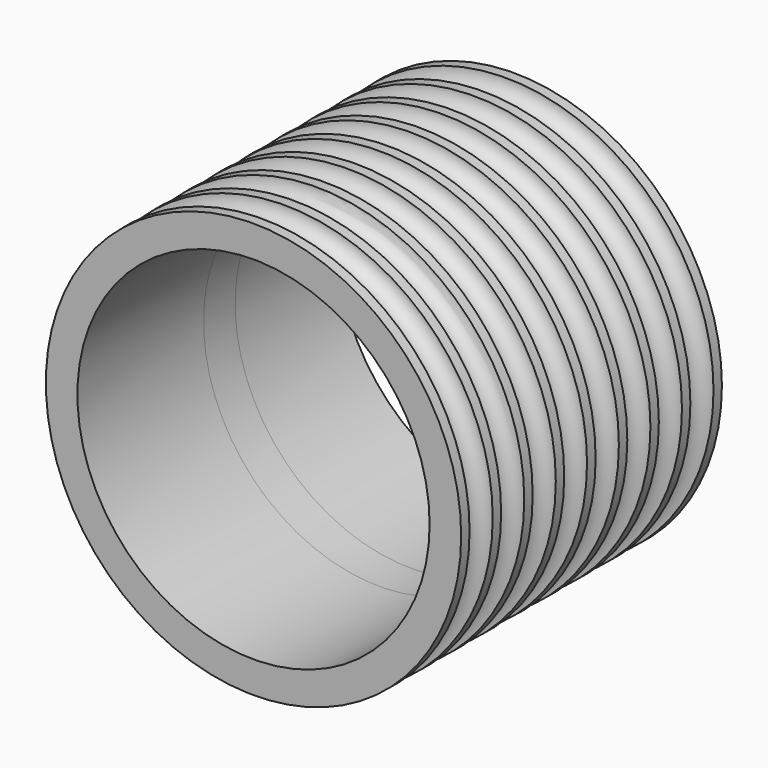
from build123d import *


# Not quite as in the source:
# - a feature names something its author has since deleted; it is built from what else it names


with BuildPart() as f1:
    # F0 (on Top) → F1 (revolve)
    with BuildSketch(Plane.XY):
        with BuildLine():
            Line((19.7205603719, 0.4943568721), (16.75, 0.4943568721))
            Line((16.75, 0.4943568721), (16.75, 0))
            Line((16.75, 0), (16.75, -2.2556431279))
            Line((16.75, -2.2556431279), (19.6911373127, -2.2556431279))
            ThreePointArc((19.6911373127, -2.2556431279), (18.3454816726, -0.8660881593), (19.7205603719, 0.4943568721))
        make_face()
        with BuildLine():
            Line((16.7490182523, 4.2443567436), (16.75, 0.4943568721))
            Line((16.75, 0.4943568721), (19.7205603719, 0.4943568721))
            Line((19.7205603719, 0.4943568721), (19.7389115558, 1.4941884749))
            ThreePointArc((19.7389115558, 1.4941884749), (18.3735909849, 2.8624558945), (19.7251108834, 4.2443567436))
            Line((19.7251108834, 4.2443567436), (16.7490182523, 4.2443567436))
        make_face()
        with BuildLine():
            Line((16.7490182523, 7.9943567436), (16.7490182523, 4.2443567436))
            Line((16.7490182523, 4.2443567436), (19.7251108834, 4.2443567436))
            ThreePointArc((19.7251108834, 4.2443567436), (19.7369436677, 4.244509486), (19.7487773282, 4.2445604014))
            Line((19.7487773282, 4.2445604014), (19.7487773282, 5.2443567436))
            ThreePointArc((19.7487773282, 5.2443567436), (18.3737773282, 6.6193567436), (19.7487773282, 7.9943567436))
            Line((19.7487773282, 7.9943567436), (16.7490182523, 7.9943567436))
        make_face()
        with BuildLine():
            Line((19.6911373127, -2.2556431279), (16.75, -2.2556431279))
            Line((16.75, -2.2556431279), (16.75, -6.0056431279))
            Line((16.75, -6.0056431279), (19.7499834311, -6.0056431279))
            ThreePointArc((19.7499834311, -6.0056431279), (18.3969368426, -4.6306431279), (19.7499834311, -3.2556431279))
            Line((19.7499834311, -3.2556431279), (19.7499834311, -2.2556431279))
            ThreePointArc((19.7499834311, -2.2556431279), (19.7205603719, -2.2559579339), (19.6911373127, -2.2556431279))
        make_face()
        with BuildLine():
            Line((19.7499834311, -2.2556431279), (19.6911373127, -2.2556431279))
            ThreePointArc((19.6911373127, -2.2556431279), (19.7205603719, -2.2559579339), (19.7499834311, -2.2556431279))
        make_face()
        with BuildLine():
            ThreePointArc((19.7487773282, 4.2445604014), (19.7369436677, 4.244509486), (19.7251108834, 4.2443567436))
            Line((19.7251108834, 4.2443567436), (19.7487773282, 4.2443567436))
            Line((19.7487773282, 4.2443567436), (19.7487773282, 4.2445604014))
        make_face()
        with BuildLine():
            Line((16.7490182523, 11.7443567436), (16.7490182523, 7.9943567436))
            Line((16.7490182523, 7.9943567436), (19.7487773282, 7.9943567436))
            Line((19.7487773282, 7.9943567436), (19.7487773282, 8.9943567436))
            ThreePointArc((19.7487773282, 8.9943567436), (18.3737773282, 10.3693567436), (19.7487773282, 11.7443567436))
            Line((19.7487773282, 11.7443567436), (16.7490182523, 11.7443567436))
        make_face()
        with BuildLine():
            Line((19.7499834311, -6.0056431279), (16.75, -6.0056431279))
            Line((16.75, -6.0056431279), (16.75, -9.7556431279))
            Line((16.75, -9.7556431279), (19.68689503, -9.7556431279))
            ThreePointArc((19.68689503, -9.7556431279), (18.3434392305, -8.3490989274), (19.7499834311, -7.0056431279))
            Line((19.7499834311, -7.0056431279), (19.7499834311, -6.0056431279))
        make_face()
        with BuildLine():
            Line((16.7490182523, 16.4943567436), (16.7490182523, 11.7443567436))
            Line((16.7490182523, 11.7443567436), (19.7487773282, 11.7443567436))
            Line((19.7487773282, 11.7443567436), (19.7487773282, 12.7443567436))
            ThreePointArc((19.7487773282, 12.7443567436), (18.3573625608, 14.1193567436), (19.7487773282, 15.4943567436))
            Line((19.7487773282, 15.4943567436), (19.7487773282, 16.4943567436))
            Line((19.7487773282, 16.4943567436), (16.7490182523, 16.4943567436))
        make_face()
        with BuildLine():
            Line((19.68689503, -9.7556431279), (16.75, -9.7556431279))
            Line((16.75, -9.7556431279), (16.75, -14.5056431279))
            Line((16.75, -14.5056431279), (19.75, -14.5056431279))
            Line((19.75, -14.5056431279), (19.75, -13.5056431279))
            ThreePointArc((19.75, -13.5056431279), (18.3547805949, -12.1306515341), (19.7499834311, -10.7556431279))
            Line((19.7499834311, -10.7556431279), (19.7499834311, -9.7556431279))
            ThreePointArc((19.7499834311, -9.7556431279), (19.7184392305, -9.7560049118), (19.68689503, -9.7556431279))
        make_face()
        with BuildLine():
            Line((19.7499834311, -9.7556431279), (19.68689503, -9.7556431279))
            ThreePointArc((19.68689503, -9.7556431279), (19.7184392305, -9.7560049118), (19.7499834311, -9.7556431279))
        make_face()
    revolve(axis=Axis((0, 3.8036210462, 0), (0, 1, 0)))


solid = f1.part
